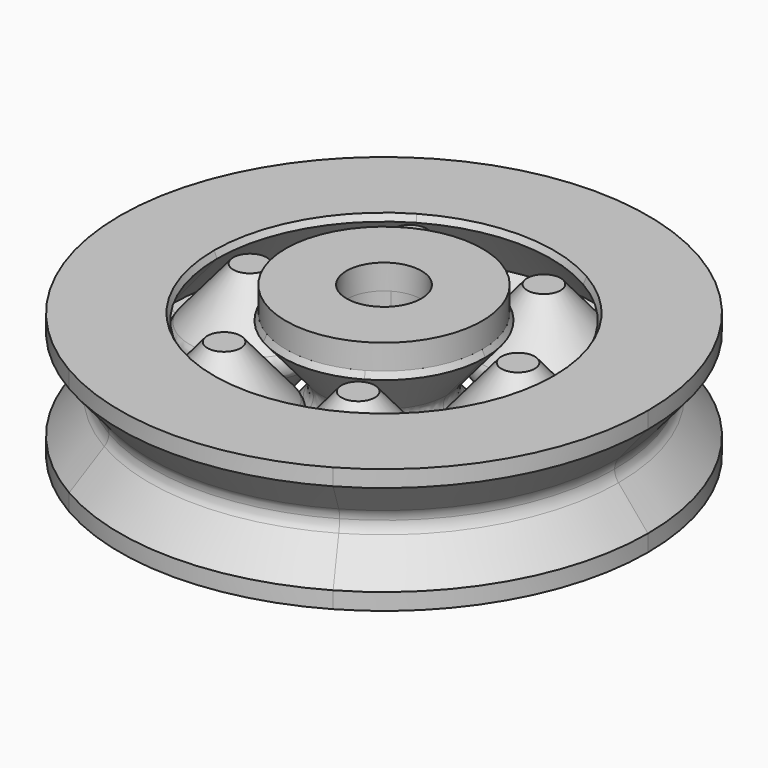
from build123d import *
from build123d import SkipClean  # not in build123d's __all__

# Parameters (mm, degrees)
F7_R      = 2
F8_COUNT  = 6
F8_ANGLE  = 300
F9_SIZE   = 1
F9_2_SIZE = 1
F9_3_SIZE = 1
F9_4_SIZE = 1
F9_5_SIZE = 1
F9_6_SIZE = 1
F10_DEPTH = 3


# Not quite as in the source:
# - after a boolean that leaves OpenCascade's solid faulty, fix() repairs it


with BuildPart() as f4:
    # F3 (on Front) → F4 (revolve)
    with BuildSketch(Plane.XZ):
        with BuildLine():
            Line((-25.6888422607, 0), (-19.3998284197, 7.4949548389))
            Line((-19.3998284197, 7.4949548389), (-31.6888422607, 7.4949548389))
            Line((-31.6888422607, 7.4949548389), (-31.6888422607, 5.4949548389))
            Line((-31.6888422607, 5.4949548389), (-28.1567533745, 1.2855752194))
            ThreePointArc((-28.1567533745, 1.2855752194), (-27.8094570191, 0.6840402867), (-27.6888422607, 0))
            Line((-27.6888422607, 0), (-25.6888422607, 0))
        make_face()
    revolve(axis=Axis((0, 0, 0), (0, 0, -1)))



with BuildPart() as f4b:
    # F3 (on Front) → F4, piece 2 (revolve)
    with BuildSketch(Plane.XZ):
        Polygon((-12.789013841, 7.4949548389), (-6.5, 0), (-4.5, 0), (-4.5, 7.4949548389), align=None)
    revolve(axis=Axis((0, 0, 0), (0, 0, -1)))


with BuildPart() as f5:
    # F3 (on Front) → F5 (revolve)
    with BuildSketch(Plane.XZ):
        Polygon((-24.3834349714, 0), (-16.0944211304, 0), (-16.0944211304, 7.4949548389), (-18.0944211304, 7.4949548389), align=None)
    revolve(axis=Axis((-16.0944211304, 0, 3.7474774195), (0, 0, -1)))


with BuildPart() as f4_1:
    add(f4.part, clean=False)

    with SkipClean():  # cleaning this boolean's faces spoils the solid; the shape is the same uncleaned
        add(f4b.part)  # F6 merges F4b

    with SkipClean():  # cleaning this boolean's faces spoils the solid; the shape is the same uncleaned
        add(f5.part)  # F6 merges F5
    # F6: F4b, F4, F5 across face
    with SkipClean():  # cleaning this boolean's faces spoils the solid; the shape is the same uncleaned
        add(f4b.part.mirror(Plane(origin=(0, 0, 0), x_dir=(1, 0, 0), z_dir=(0, 0, -1))), clean=False)
        add(f4.part.mirror(Plane(origin=(0, 0, 0), x_dir=(1, 0, 0), z_dir=(0, 0, -1))), clean=False)
        add(f5.part.mirror(Plane(origin=(0, 0, 0), x_dir=(1, 0, 0), z_dir=(0, 0, -1))), clean=False)

    add(f4_1.part.fix(), mode=Mode.REPLACE)

    # F7
    f7_edges = [f4_1.edges().sort_by_distance(p)[0] for p in [
        (-7.805407, 0, 0),
        (6.5, 0, 0),
    ]]
    fillet(f7_edges, radius=F7_R)


with BuildPart() as f8_1:
    # F8: instance of F4
    add(f4_1.part.rotate(Axis((0, 0, 0), (0, 0, -1)), 1 * F8_ANGLE / (F8_COUNT - 1)), clean=False)

    # F9#2
    f9_2_edges = [f8_1.edges().sort_by_distance(p)[0] for p in [
        (6.394507, -11.075611, 7.494955),
        (6.394507, -11.075611, -7.494955),
        (9.699914, -16.800744, 7.494955),
        (9.699914, -16.800744, -7.494955),
    ]]
    chamfer(f9_2_edges, length=F9_2_SIZE)


with BuildPart() as f8_2:
    # F8: instance of F4
    add(f4_1.part.rotate(Axis((0, 0, 0), (0, 0, -1)), 2 * F8_ANGLE / (F8_COUNT - 1)), clean=False)

    # F9#3
    f9_3_edges = [f8_2.edges().sort_by_distance(p)[0] for p in [
        (-6.394507, -11.075611, 7.494955),
        (-6.394507, -11.075611, -7.494955),
        (-9.699914, -16.800744, 7.494955),
        (-9.699914, -16.800744, -7.494955),
    ]]
    chamfer(f9_3_edges, length=F9_3_SIZE)


with BuildPart() as f8_3:
    # F8: instance of F4
    add(f4_1.part.rotate(Axis((0, 0, 0), (0, 0, -1)), 3 * F8_ANGLE / (F8_COUNT - 1)), clean=False)

    # F9#4
    f9_4_edges = [f8_3.edges().sort_by_distance(p)[0] for p in [
        (-12.789014, 0, 7.494955),
        (-12.789014, 0, -7.494955),
        (-19.399828, 0, 7.494955),
        (-19.399828, 0, -7.494955),
    ]]
    chamfer(f9_4_edges, length=F9_4_SIZE)


with BuildPart() as f8_4:
    # F8: instance of F4
    add(f4_1.part.rotate(Axis((0, 0, 0), (0, 0, -1)), 4 * F8_ANGLE / (F8_COUNT - 1)), clean=False)

    # F9#5
    f9_5_edges = [f8_4.edges().sort_by_distance(p)[0] for p in [
        (-6.394507, 11.075611, 7.494955),
        (-6.394507, 11.075611, -7.494955),
        (-9.699914, 16.800744, 7.494955),
        (-9.699914, 16.800744, -7.494955),
    ]]
    chamfer(f9_5_edges, length=F9_5_SIZE)


with BuildPart() as f8_5:
    # F8: instance of F4
    add(f4_1.part.rotate(Axis((0, 0, 0), (0, 0, -1)), 5 * F8_ANGLE / (F8_COUNT - 1)), clean=False)

    # F9#6
    f9_6_edges = [f8_5.edges().sort_by_distance(p)[0] for p in [
        (6.394507, 11.075611, 7.494955),
        (6.394507, 11.075611, -7.494955),
        (9.699914, 16.800744, 7.494955),
        (9.699914, 16.800744, -7.494955),
    ]]
    chamfer(f9_6_edges, length=F9_6_SIZE)


with BuildPart() as f4_2:
    add(f4_1.part, clean=False)

    # F9
    f9_edges = [f4_2.edges().sort_by_distance(p)[0] for p in [
        (12.789014, 0, 7.494955),
        (19.399828, 0, 7.494955),
        (19.399828, 0, -7.494955),
        (12.789014, 0, -7.494955),
    ]]
    chamfer(f9_edges, length=F9_SIZE)

    # F10 (add): a face of the model
    f10_faces = [f4_2.faces().sort_by_distance(p)[0] for p in [
        (11.4555701758, 0, 7.4949548389),
    ]]

    with SkipClean():  # cleaning this boolean's faces spoils the solid; the shape is the same uncleaned
        add(f8_1.part)  # F10 merges F8_1

    with SkipClean():  # cleaning this boolean's faces spoils the solid; the shape is the same uncleaned
        add(f8_2.part)  # F10 merges F8_2

    with SkipClean():  # cleaning this boolean's faces spoils the solid; the shape is the same uncleaned
        add(f8_3.part)  # F10 merges F8_3

    with SkipClean():  # cleaning this boolean's faces spoils the solid; the shape is the same uncleaned
        add(f8_4.part)  # F10 merges F8_4

    with SkipClean():  # cleaning this boolean's faces spoils the solid; the shape is the same uncleaned
        add(f8_5.part)  # F10 merges F8_5
    with SkipClean():  # cleaning this boolean's faces spoils the solid; the shape is the same uncleaned
        extrude(f10_faces, amount=F10_DEPTH)


solid = f4_2.part
